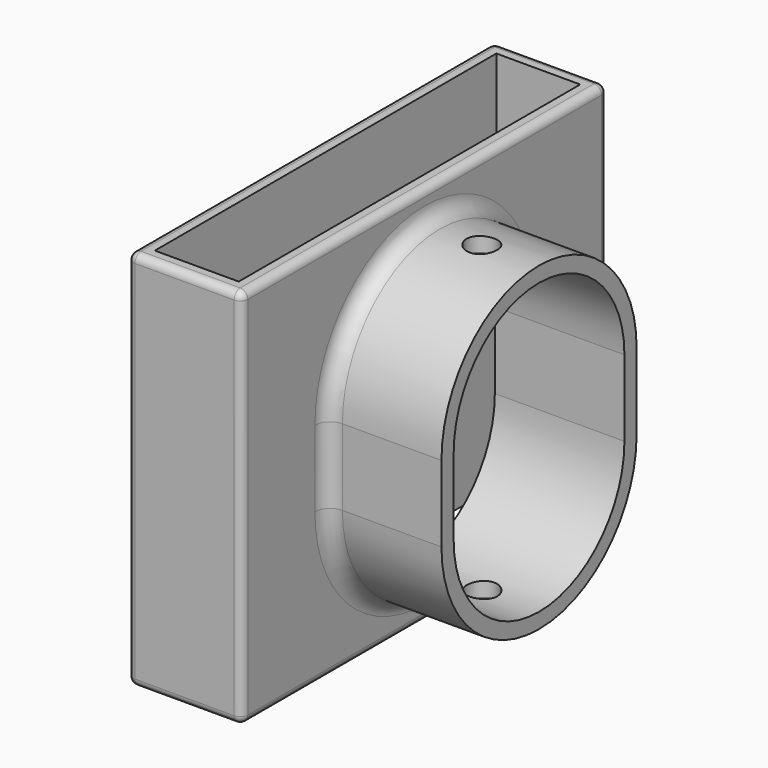
from build123d import *

# Parameters (mm, degrees)
F3_W     = 3810
F3_H     = 15240
F3_W_2   = 2794
F3_H_2   = 14224
F4_DEPTH = 5080
F6_DEPTH = 3810
F7_DEPTH = 508
F9_DEPTH = 1270
F10_R    = 254
F14_D    = 1016
F16_R    = 508


# Not quite as in the source:
# - a variable given as a bare number and used for a length is read in inches; the dataset says mm whatever the document's units were


with BuildPart() as f4:
    # F3 (on Top) → F4 (new body)
    with BuildSketch(Plane.XY):
        Rectangle(F3_W, F3_H)
        Rectangle(F3_W_2, F3_H_2, mode=Mode.SUBTRACT)
    extrude(amount=F4_DEPTH)

    # F5 (on face) → F6 (join)
    with BuildSketch(Plane.YZ.offset(1905)):
        with BuildLine():
            Line((3556, 0), (4064, 0))
            ThreePointArc((4064, 0), (0, 4064), (-4064, 0))
            Line((-4064, 0), (-3556, 0))
            ThreePointArc((-3556, 0), (0, 3556), (3556, 0))
        make_face()
    extrude(amount=F6_DEPTH)

    # F7 (cut, through all): a face of the model
    f7_faces = [f4.faces().sort_by_distance(p)[0] for p in [
        (1905, 0, 1509.2132736927),
    ]]
    extrude(f7_faces, amount=-F7_DEPTH, mode=Mode.SUBTRACT)

    # F8 (on face) → F9 (join)
    with BuildSketch(Plane(origin=(0, 0, 0), x_dir=(1, 0, 0), z_dir=(0, 0, -1))):
        Polygon((1905, 4064), (1905, 7620), (-1905, 7620), (-1905, -7620), (1905, -7620), (1905, -4064), (5715, -4064), (5715, -3556), (1397, -3556), (1397, -7112), (-1397, -7112), (-1397, 7112), (1397, 7112), (1397, 3556), (5715, 3556), (5715, 4064), align=None)
    extrude(amount=F9_DEPTH)

    # F10
    f10_edges = [f4.edges().sort_by_distance(p)[0] for p in [
        (0, -7620, 5080),
        (1905, 0, 5080),
        (0, 7620, 5080),
        (-1905, 0, 5080),
        (1905, -7620, 1905),
        (1905, 7620, 1905),
        (-1905, -7620, 1905),
        (-1905, 7620, 1905),
    ]]
    fillet(f10_edges, radius=F10_R)

    # F14 (through all)
    with Locations(Plane.XY.offset(4064)):
        with Locations((3810, 0)):
            Hole(F14_D / 2)

    # F15: F4 across face


with BuildPart() as f4_1:
    add(f4.part)
    add(f4.part.mirror(Plane(origin=(474.1354212806, 0, -1270), x_dir=(1, 0, 0), z_dir=(0, 0, -1))))

    # F16
    f16_edges = [f4_1.edges().sort_by_distance(p)[0] for p in [
        (1905, -7366, -1270),
        (1905, 0, 4826),
        (1905, 7366, -1270),
        (1905, 0, -7366),
        (1905, -4064, -1270),
        (1905, 0, -6604),
        (1905, 4064, -1270),
        (1905, 0, 4064),
    ]]
    fillet(f16_edges, radius=F16_R)


solid = f4_1.part
